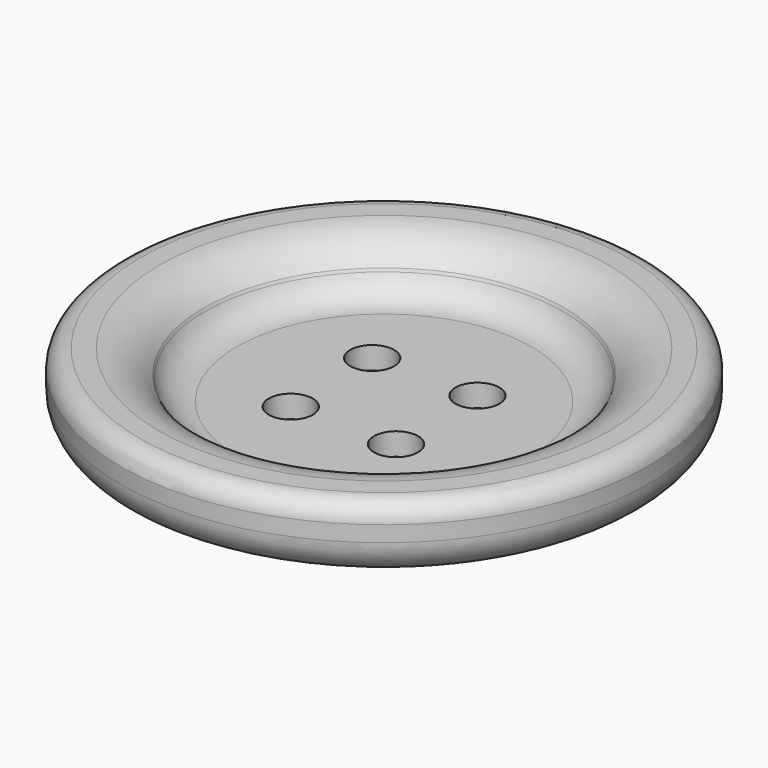
from build123d import *

# Parameters (mm, degrees)
F2_R     = 1.25
F3_DEPTH = 5.1


# Not quite as in the source:
# - a feature names something its author has since deleted; it is built from what else it names


with BuildPart() as f1:
    # F0 (on Front) → F1 (revolve)
    with BuildSketch(Plane.XZ):
        with BuildLine():
            Line((0, 1.2750519672), (0, 0))
            Line((0, 0), (13, 0))
            ThreePointArc((13, 0), (14.4142135624, 0.5857864376), (15, 2))
            Line((15, 2), (15, 2.8974551242))
            ThreePointArc((15, 2.8974551242), (14.6395651733, 3.6234077181), (13.8866530545, 3.9234806662))
            Line((13.8866530545, 3.9234806662), (12.773306109, 3.9234806662))
            ThreePointArc((12.773306109, 3.9234806662), (11.3706801368, 3.5459784592), (10.2690433302, 2.5992663167))
            Line((10.2690433302, 2.5992663167), (10.1940094677, 2.4367391619))
            ThreePointArc((10.1940094677, 2.4367391619), (9.4559973183, 1.5903226699), (8.378181381, 1.2750519672))
            Line((8.378181381, 1.2750519672), (0, 1.2750519672))
        make_face()
    revolve(axis=Axis((0, 0, 0.6375259836), (0, 0, -1)))

    # F2 (on face) → F3 (cut)
    with BuildSketch(Plane.XY.offset(1.2750519672)):
        with Locations((3.0000000261, -2.9038460925)):
            Circle(F2_R)
        with Locations((2.9038460925, 3.0000000261)):
            Circle(F2_R)
        with Locations((-3.0000000261, 2.9038460925)):
            Circle(F2_R)
        with Locations((-2.9038460925, -3.0000000261)):
            Circle(F2_R)
    extrude(amount=-F3_DEPTH, mode=Mode.SUBTRACT)


solid = f1.part
